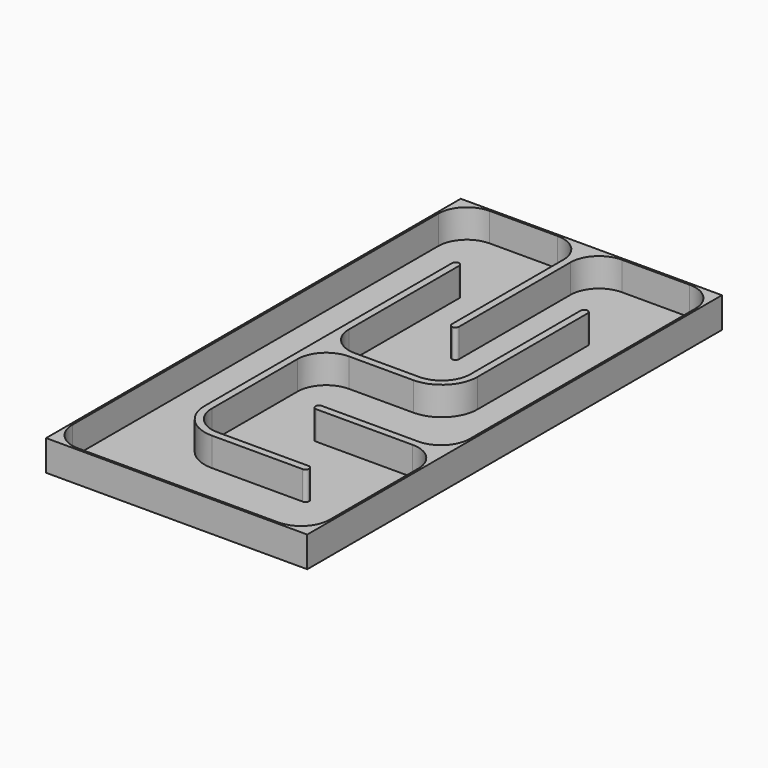
from build123d import *

# Parameters (mm, degrees)
F6_W          = 1828
F6_H          = 3628
F7_DEPTH      = 14
F7_DEPTH_BACK = 200
F8_T          = -14
F14_W         = 50
F14_H         = 200
F13_W         = 50
F13_H         = 200
F12_W         = 50
F12_H         = 200
F20_R         = 200
F20_2_R       = 200
F21_R         = 24.99999
F21_2_R       = 24.99999
F22_R         = 250


# Not quite as in the source:
# - a fillet or chamfer is up to 0.001 mm smaller than in the source, because OpenCascade refuses the exact size


with BuildPart() as f7:
    # F6 (on Top) → F7 (new body, two sides)
    with BuildSketch(Plane.XY) as f7_sk:
        Rectangle(F6_W, F6_H)
    extrude(amount=-F7_DEPTH)
    extrude(f7_sk.sketch, amount=F7_DEPTH_BACK)

    # F8
    f8_openings = [f7.faces().sort_by_distance(p)[0] for p in [
        (0, 0, 200),
    ]]
    offset(amount=F8_T, openings=f8_openings)

    # F15: sweep along a path in F9
    with BuildLine(Plane.XY) as f15_path:
        Line((0, -600), (900, -600))
    # F14 (on Right) → F15 (sweep)
    with BuildSketch(Plane.YZ):
        with Locations((-600, 100)):
            Rectangle(F14_W, F14_H)
    sweep(path=f15_path.line)

    # F17: sweep along a path in F9
    with BuildLine(Plane.XY) as f17_path:
        Line((0, 1800), (0, 600))
    # F12 (on plane+point) → F17 (sweep)
    with BuildSketch(Plane.XZ.offset(-600)):
        with Locations((0, 100)):
            Rectangle(F12_W, F12_H)
    sweep(path=f17_path.line)

    # F20
    f20_edges = [f7.edges().sort_by_distance(p)[0] for p in [
        (25, 1800, 100),
        (900, 1800, 100),
        (-25, 1800, 100),
        (-900, 1800, 100),
        (-900, -1800, 100),
        (900, -575, 100),
        (900, -625, 100),
        (900, -1800, 100),
    ]]
    fillet(f20_edges, radius=F20_R)

    # F21 (radius 25 in the source; OpenCascade refuses exactly that, so slightly less here)
    f21_edges = [f7.edges().sort_by_distance(p)[0] for p in [
        (-25, 600, 100),
        (25, 600, 100),
        (0, -575, 100),
        (0, -625, 100),
    ]]
    fillet(f21_edges, radius=F21_R)


with BuildPart() as f16:
    # F16: sweep along a path in F9
    with BuildLine(Plane.XY) as f16_path:
        Line((-450, 1200), (-450, -1200))
        Line((-450, -1200), (450, -1200))
    # F13 (on offset) → F16 (sweep)
    with BuildSketch(Plane(origin=(0, 1214, 0), x_dir=(-1, 0, 0), z_dir=(0, 1, 0))):
        with Locations((450, 100)):
            Rectangle(F13_W, F13_H)
    sweep(path=f16_path.line, transition=Transition.RIGHT)

    # F18: sweep along a path in F9
    with BuildLine(Plane.XY) as f18_path:
        Line((450, 1200), (450, 0))
        Line((450, 0), (-450, 0))
    # F13 (on offset) → F18 (sweep)
    with BuildSketch(Plane(origin=(0, 1214, 0), x_dir=(-1, 0, 0), z_dir=(0, 1, 0))):
        with Locations((-450, 100)):
            Rectangle(F13_W, F13_H)
    sweep(path=f18_path.line, transition=Transition.RIGHT)

    # F19: union 

    # F20#2
    f20_2_edges = [f16.edges().sort_by_distance(p)[0] for p in [
        (-425, -1175, 100),
        (425, 25, 100),
        (-425, 25, 100),
        (-425, -25, 100),
    ]]
    fillet(f20_2_edges, radius=F20_2_R)

    # F21#2 (radius 25 in the source; OpenCascade refuses exactly that, so slightly less here)
    f21_2_edges = [f16.edges().sort_by_distance(p)[0] for p in [
        (436, -1175, 100),
        (436, -1225, 100),
        (425, 1214, 100),
        (475, 1214, 100),
        (-475, 1214, 100),
        (-425, 1214, 100),
    ]]
    fillet(f21_2_edges, radius=F21_2_R)

    # F22
    f22_edges = [f16.edges().sort_by_distance(p)[0] for p in [
        (475, -25, 100),
        (-475, -1225, 100),
    ]]
    fillet(f22_edges, radius=F22_R)


solid = Compound([f7.part, f16.part])
